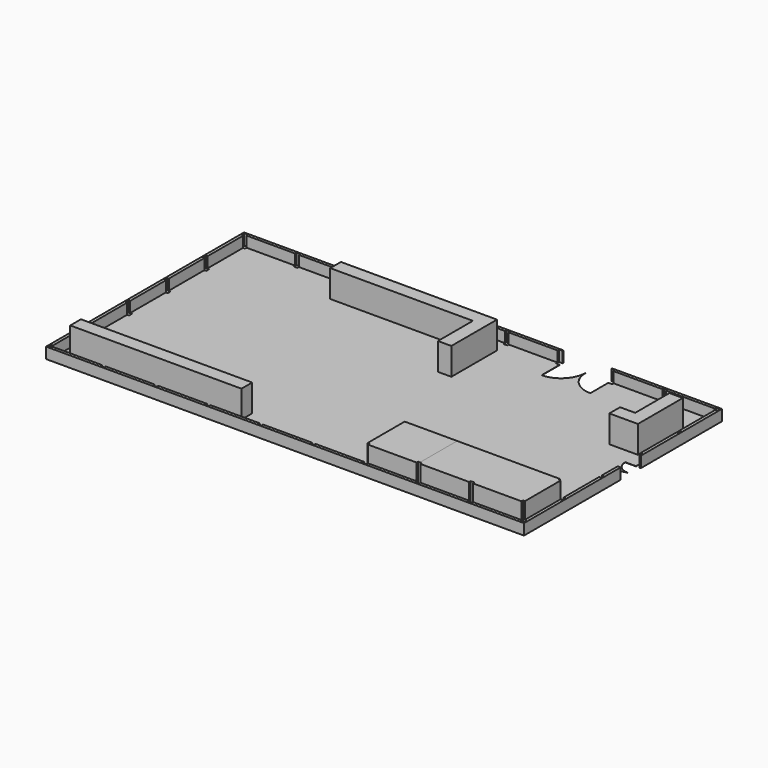
from build123d import *

# Parameters (mm, degrees)
F0_W     = 15600
F0_H     = 1220
F1_DEPTH = 25
F0_W_2   = 13000
F2_DEPTH = 2500
F0_W_3   = 1220
F0_H_2   = 3900
F3_DEPTH = 2500
F4_DEPTH = 1000


with BuildPart() as f1:
    # F0 (on Top) → F1 (new body)
    with BuildSketch(Plane.XY):
        Polygon((28666.6668, 170), (28666.6668, 4400), (28666.6668, 10000), (0, 10000), (0, 8970), (170, 8970), (170, 8630), (0, 8630), (0, 4570), (170, 4570), (170, 4230), (0, 4230), (0, 170), (170, 170), (170, 0), (4607.7778, 0), (4607.7778, 170), (4947.7778, 170), (4947.7778, 0), (9385.5556, 0), (9385.5556, 170), (9725.5556, 170), (9725.5556, 0), (14163.3334, 0), (14163.3334, 170), (14503.3334, 170), (14503.3334, 0), (18941.1112, 0), (18941.1112, 170), (19281.1112, 170), (19281.1112, 0), (23718.889, 0), (23718.889, 170), (24058.889, 170), (24058.889, 0), (28496.6668, 0), (28496.6668, 170), align=None)
        with Locations((8633.9790344238, 1710.9863615036)):
            Rectangle(F0_W, F0_H, mode=Mode.SUBTRACT)
        with BuildLine():
            ThreePointArc((33274.4446, 19781.1111), (31705.4532121104, 20431.0086121104), (31055.5557, 22000))
            ThreePointArc((31055.5557, 22000), (30405.6581878896, 20431.0086121104), (28836.6668, 19781.1111))
            Line((28836.6668, 19781.1111), (28836.6668, 21830))
            Line((28836.6668, 21830), (28496.6668, 21830))
            Line((28496.6668, 21830), (28496.6668, 22000))
            Line((28496.6668, 22000), (24058.889, 22000))
            Line((24058.889, 22000), (24058.889, 21830))
            Line((24058.889, 21830), (23718.889, 21830))
            Line((23718.889, 21830), (23718.889, 22000))
            Line((23718.889, 22000), (19281.1112, 22000))
            Line((19281.1112, 22000), (19281.1112, 21830))
            Line((19281.1112, 21830), (18941.1112, 21830))
            Line((18941.1112, 21830), (18941.1112, 22000))
            Line((18941.1112, 22000), (14503.3334, 22000))
            Line((14503.3334, 22000), (14503.3334, 21830))
            Line((14503.3334, 21830), (14163.3334, 21830))
            Line((14163.3334, 21830), (14163.3334, 22000))
            Line((14163.3334, 22000), (9725.5556, 22000))
            Line((9725.5556, 22000), (9725.5556, 21830))
            Line((9725.5556, 21830), (9385.5556, 21830))
            Line((9385.5556, 21830), (9385.5556, 22000))
            Line((9385.5556, 22000), (4947.7778, 22000))
            Line((4947.7778, 22000), (4947.7778, 21830))
            Line((4947.7778, 21830), (4607.7778, 21830))
            Line((4607.7778, 21830), (4607.7778, 22000))
            Line((4607.7778, 22000), (170, 22000))
            Line((170, 22000), (170, 21830))
            Line((170, 21830), (0, 21830))
            Line((0, 21830), (0, 17770))
            Line((0, 17770), (170, 17770))
            Line((170, 17770), (170, 17430))
            Line((170, 17430), (0, 17430))
            Line((0, 17430), (0, 13370))
            Line((0, 13370), (170, 13370))
            Line((170, 13370), (170, 13030))
            Line((170, 13030), (0, 13030))
            Line((0, 13030), (0, 12000))
            Line((0, 12000), (0, 10000))
            Line((0, 10000), (28666.6668, 10000))
            Line((28666.6668, 10000), (28666.6668, 4400))
            Line((28666.6668, 4400), (33444.4446, 4400))
            Line((33444.4446, 4400), (42830, 4400))
            Line((42830, 4400), (42830, 4570))
            Line((42830, 4570), (43000, 4570))
            Line((43000, 4570), (43000, 8630))
            Line((43000, 8630), (42830, 8630))
            Line((42830, 8630), (42830, 8970))
            Line((42830, 8970), (43000, 8970))
            Line((43000, 8970), (43000, 10730))
            Line((43000, 10730), (41850, 10730))
            ThreePointArc((41850, 10730), (42186.8272016355, 11543.1727983645), (43000, 11880))
            ThreePointArc((43000, 11880), (42186.8272016355, 12216.8272016355), (41850, 13030))
            Line((41850, 13030), (42830, 13030))
            Line((42830, 13030), (42830, 13370))
            Line((42830, 13370), (43000, 13370))
            Line((43000, 13370), (43000, 17430))
            Line((43000, 17430), (42830, 17430))
            Line((42830, 17430), (42830, 17770))
            Line((42830, 17770), (43000, 17770))
            Line((43000, 17770), (43000, 21830))
            Line((43000, 21830), (42830.0002, 21830))
            Line((42830.0002, 21830), (42830.0002, 22000))
            Line((42830.0002, 22000), (38392.2224, 22000))
            Line((38392.2224, 22000), (38392.2224, 21830))
            Line((38392.2224, 21830), (38052.2224, 21830))
            Line((38052.2224, 21830), (38052.2224, 22000))
            Line((38052.2224, 22000), (33614.4446, 22000))
            Line((33614.4446, 22000), (33614.4446, 21830))
            Line((33614.4446, 21830), (33274.4446, 21830))
            Line((33274.4446, 21830), (33274.4446, 19781.1111))
        make_face()
        Polygon((9758.5079956055, 19549.7811126709), (9758.5079956055, 20769.7811126709), (22758.5079956055, 20769.7811126709), (23978.5079956055, 20769.7811126709), (23978.5079956055, 15569.7811126709), (22758.5079956055, 15569.7811126709), (22758.5079956055, 19549.7811126709), align=None, mode=Mode.SUBTRACT)
        Polygon((39250, 14475.3923416138), (39250, 15695.3923416138), (40630, 15695.3923416138), (40630, 19595.3923416138), (41850, 19595.3923416138), (41850, 15695.3923416138), (41850, 14475.3923416138), align=None, mode=Mode.SUBTRACT)
    extrude(amount=F1_DEPTH)

    # F0 (on Top) → F4 (join)
    with BuildSketch(Plane.XY):
        Polygon((24058.889, 22000), (28496.6668, 22000), (28496.6668, 22170), (28836.6668, 22170), (28836.6668, 22270), (-270, 22270), (-270, -270), (43270.0002, -270), (43270.0002, 10730), (43000, 10730), (43000, 8970), (43170, 8970), (43170, 8630), (43000, 8630), (43000, 4570), (43170, 4570), (43170, 4230), (43000.0000077273, 4230), (43000.0001922727, 170), (43170.0002, 170), (43170.0002, -170), (42830.0002, -170), (42830.0002, 0), (38392.2224, 0), (38392.2224, -170), (38052.2224, -170), (38052.2224, 0), (33614.4446, 0), (33614.4446, -170), (33274.4446, -170), (33274.4446, 0), (28836.6668, 0), (28836.6668, -170), (28496.6668, -170), (28496.6668, 0), (24058.889, 0), (24058.889, -170), (23718.889, -170), (23718.889, 0), (19281.1112, 0), (19281.1112, -170), (18941.1112, -170), (18941.1112, 0), (14503.3334, 0), (14503.3334, -170), (14163.3334, -170), (14163.3334, 0), (9725.5556, 0), (9725.5556, -170), (9385.5556, -170), (9385.5556, 0), (4947.7778, 0), (4947.7778, -170), (4607.7778, -170), (4607.7778, 0), (170, 0), (170, -170), (-170, -170), (-170, 170), (0, 170), (0, 4230), (-170, 4230), (-170, 4570), (0, 4570), (0, 8630), (-170, 8630), (-170, 8970), (0, 8970), (0, 10000), (0, 12000), (0, 13030), (-170, 13030), (-170, 13370), (0, 13370), (0, 17430), (-170, 17430), (-170, 17770), (0, 17770), (0, 21830), (-170, 21830), (-170, 22170), (170, 22170), (170, 22000), (4607.7778, 22000), (4607.7778, 22170), (4947.7778, 22170), (4947.7778, 22000), (9385.5556, 22000), (9385.5556, 22170), (9725.5556, 22170), (9725.5556, 22000), (14163.3334, 22000), (14163.3334, 22170), (14503.3334, 22170), (14503.3334, 22000), (18941.1112, 22000), (18941.1112, 22170), (19281.1112, 22170), (19281.1112, 22000), (23718.889, 22000), (23718.889, 22170), (24058.889, 22170), align=None)
        Polygon((33614.4446, 22170), (33614.4446, 22000), (38052.2224, 22000), (38052.2224, 22170), (38392.2224, 22170), (38392.2224, 22000), (42830.0002, 22000), (42830.0002, 22170), (43170.0002, 22170), (43170.0002, 21830), (43000, 21830), (43000, 17770), (43170, 17770), (43170, 17430), (43000, 17430), (43000, 13370), (43170, 13370), (43170, 13030), (43270.0002, 13030), (43270.0002, 22270), (33274.4446, 22270), (33274.4446, 22170), align=None)
    extrude(amount=F4_DEPTH)


with BuildPart() as f2:
    # F0 (on Top) → F2 (new body)
    with BuildSketch(Plane.XY):
        with Locations((16258.5079956055, 20159.7811126709)):
            Rectangle(F0_W_2, F0_H)
        Polygon((23978.5079956055, 20769.7811126709), (22758.5079956055, 20769.7811126709), (22758.5079956055, 19549.7811126709), (22758.5079956055, 15569.7811126709), (23978.5079956055, 15569.7811126709), align=None)
    extrude(amount=F2_DEPTH)


with BuildPart() as f2b:
    # F0 (on Top) → F2, piece 2 (new body)
    with BuildSketch(Plane.XY):
        with Locations((8633.9790344238, 1710.9863615036)):
            Rectangle(F0_W, F0_H)
    extrude(amount=F2_DEPTH)


with BuildPart() as f2c:
    # F0 (on Top) → F2, piece 3 (new body)
    with BuildSketch(Plane.XY):
        with Locations((41240, 17645.3923416138)):
            Rectangle(F0_W_3, F0_H_2)
        Polygon((40630, 15695.3923416138), (39250, 15695.3923416138), (39250, 14475.3923416138), (41850, 14475.3923416138), (41850, 15695.3923416138), align=None)
    extrude(amount=F2_DEPTH)


with BuildPart() as f2d:
    # F0 (on Top) → F2, piece 4 (new body)
    with BuildSketch(Plane.XY):
        Polygon((43000.0001922727, 170), (43000.0000077273, 4230), (42830, 4230), (42830, 4400), (33444.4446, 4400), (33444.4446, 170), (33614.4446, 170), (33614.4446, 0), (38052.2224, 0), (38052.2224, 170), (38392.2224, 170), (38392.2224, 0), (42830.0002, 0), (42830.0002, 170), align=None)
    extrude(amount=F2_DEPTH)


with BuildPart() as f3:
    # F0 (on Top) → F3 (new body)
    with BuildSketch(Plane.XY):
        Polygon((33444.4446, 170), (33444.4446, 4400), (28666.6668, 4400), (28666.6668, 170), (28836.6668, 170), (28836.6668, 0), (33274.4446, 0), (33274.4446, 170), align=None)
    extrude(amount=F3_DEPTH)


solid = Compound([f1.part, f2.part, f2b.part, f2c.part, f2d.part, f3.part])
